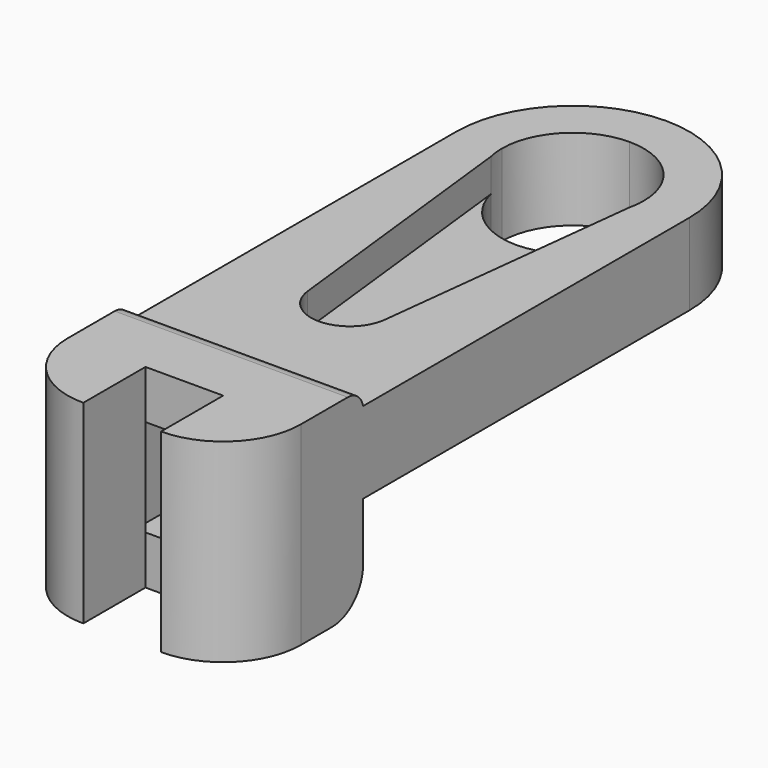
from build123d import *

# Parameters (mm, degrees)
F1_DEPTH      = 4.2
F2_DEPTH      = 2.5
F3_DEPTH      = 5
F3_DEPTH_BACK = 5
F4_W          = 5
F4_H          = 5
F5_DEPTH      = 4
F5_DEPTH_BACK = 4
F6_SIZE       = 2
F7_W          = 4
F7_H          = 2.5
F8_DEPTH      = 25
F9_R          = 2
F11_DEPTH     = 1
F13_DEPTH     = 1
F14_T1_DEPTH  = 16.8989794856


# Not quite as in the source:
# - a fillet or chamfer that OpenCascade refuses, or shapes differently, is made with other operations: its cross-section is extruded or revolved along the edge and cut away or added


with BuildPart() as f1:
    # F0 (on Top) → F1 (new body)
    with BuildSketch(Plane.XY):
        with BuildLine():
            ThreePointArc((6, 14.5), (0, 20.5), (-6, 14.5))
            Line((-6, 14.5), (-3.65, 14.5))
            ThreePointArc((-3.65, 14.5), (-2.5809397513, 17.0809397513), (0, 18.15))
            ThreePointArc((0, 18.15), (2.5809397513, 17.0809397513), (3.65, 14.5))
            Line((3.65, 14.5), (6, 14.5))
        make_face()
        with BuildLine():
            Line((6, -6.5), (-6, -6.5))
            Line((-6, -6.5), (-6, -10.5))
            ThreePointArc((-6, -10.5), (-4.8284271247, -13.3284271247), (-2, -14.5))
            Line((-2, -14.5), (-2, -10.5))
            Line((-2, -10.5), (0, -10.5))
            Line((0, -10.5), (2, -10.5))
            Line((2, -10.5), (2, -14.5))
            ThreePointArc((2, -14.5), (4.8284271247, -13.3284271247), (6, -10.5))
            Line((6, -10.5), (6, -6.5))
        make_face()
        with BuildLine():
            Line((-3.65, 14.5), (-6, 14.5))
            Line((-6, 14.5), (-6, -6.5))
            Line((-6, -6.5), (6, -6.5))
            Line((6, -6.5), (6, 14.5))
            Line((6, 14.5), (3.65, 14.5))
            ThreePointArc((3.65, 14.5), (3.6264789057, 14.0862963062), (3.5562187692, 13.6779245377))
            Line((3.5562187692, 13.6779245377), (1.9871117367, -0.0766868897))
            ThreePointArc((1.9871117367, -0.0766868897), (1.3316580306, -1.3422087286), (0, -1.85))
            ThreePointArc((0, -1.85), (-1.3316580225, -1.3422087358), (-1.9871117342, -0.0766869112))
            Line((-1.9871117342, -0.0766869112), (-3.5562187692, 13.6779245377))
            ThreePointArc((-3.5562187692, 13.6779245377), (-3.6264789057, 14.0862963062), (-3.65, 14.5))
        make_face()
    extrude(amount=F1_DEPTH)

    # F0 (on Top) → F2 (join)
    with BuildSketch(Plane.XY):
        with BuildLine():
            ThreePointArc((0, 10.85), (-2.2717751388, 11.6431594866), (-3.5562187692, 13.6779245377))
            Line((-3.5562187692, 13.6779245377), (-1.9871117342, -0.0766869112))
            ThreePointArc((-1.9871117342, -0.0766869112), (-1.4922087358, 1.4816580225), (0, 2.15))
            Line((0, 2.15), (0, 10.85))
        make_face()
        with BuildLine():
            ThreePointArc((3.5562187692, 13.6779245377), (2.2717751388, 11.6431594866), (0, 10.85))
            Line((0, 10.85), (0, 2.15))
            ThreePointArc((0, 2.15), (1.4142135624, 1.5642135624), (2, 0.15))
            ThreePointArc((2, 0.15), (1.9967753346, 0.0364735127), (1.9871117367, -0.0766868897))
            Line((1.9871117367, -0.0766868897), (3.5562187692, 13.6779245377))
        make_face()
        with BuildLine():
            ThreePointArc((0, 2.15), (-1.4922087358, 1.4816580225), (-1.9871117342, -0.0766869112))
            ThreePointArc((-1.9871117342, -0.0766869112), (-1.3316580225, -1.3422087358), (0, -1.85))
            Line((0, -1.85), (0, 2.15))
        make_face()
        with BuildLine():
            ThreePointArc((2, 0.15), (1.4142135624, 1.5642135624), (0, 2.15))
            Line((0, 2.15), (0, -1.85))
            ThreePointArc((0, -1.85), (1.3316580306, -1.3422087286), (1.9871117367, -0.0766868897))
            ThreePointArc((1.9871117367, -0.0766868897), (1.9967753346, 0.0364735127), (2, 0.15))
        make_face()
    extrude(amount=F2_DEPTH)

    # F0 (on Top) → F3 (join, two sides)
    with BuildSketch(Plane.XY) as f3_sk:
        with BuildLine():
            Line((6, -6.5), (-6, -6.5))
            Line((-6, -6.5), (-6, -10.5))
            ThreePointArc((-6, -10.5), (-4.8284271247, -13.3284271247), (-2, -14.5))
            Line((-2, -14.5), (-2, -10.5))
            Line((-2, -10.5), (0, -10.5))
            Line((0, -10.5), (2, -10.5))
            Line((2, -10.5), (2, -14.5))
            ThreePointArc((2, -14.5), (4.8284271247, -13.3284271247), (6, -10.5))
            Line((6, -10.5), (6, -6.5))
        make_face()
    extrude(amount=F3_DEPTH)
    extrude(f3_sk.sketch, amount=-F3_DEPTH_BACK)

    # F4 (on face) → F5 (cut, two sides)
    with BuildSketch(Plane(origin=(0, -6.5, 0), x_dir=(-1, 0, 0), z_dir=(0, 1, 0))) as f5_sk:
        Rectangle(F4_W, F4_H)
    extrude(amount=-F5_DEPTH, mode=Mode.SUBTRACT)
    extrude(f5_sk.sketch, amount=F5_DEPTH_BACK, mode=Mode.SUBTRACT)

    # F6
    f6_edges = [f1.edges().sort_by_distance(p)[0] for p in [
        (0, -2.5, 2.5),
    ]]
    chamfer(f6_edges, length=F6_SIZE)

    # F7 (on face) → F8 (cut)
    with BuildSketch(Plane.XZ.offset(10.5)):
        with Locations((0, -3.75)):
            Rectangle(F7_W, F7_H)
    extrude(amount=-F8_DEPTH, mode=Mode.SUBTRACT)

    # F9
    f9_edges = [f1.edges().sort_by_distance(p)[0] for p in [
        (4, -6.5, -5),
        (-4, -6.5, -5),
    ]]
    fillet(f9_edges, radius=F9_R)

    # F10 (on face) → F11 (join)
    with BuildSketch(Plane.YZ.offset(-2)):
        with BuildLine():
            Line((-6.5, -2.5), (-10.5, -2.5))
            Line((-10.5, -2.5), (-10.5, -5))
            Line((-10.5, -5), (-8.5, -5))
            ThreePointArc((-8.5, -5), (-7.0857864376, -4.4142135624), (-6.5, -3))
            Line((-6.5, -3), (-6.5, -2.5))
        make_face()
    extrude(amount=F11_DEPTH)

    # F12 (on face) → F13 (join)
    with BuildSketch(Plane(origin=(2, 0, 0), x_dir=(0, -1, 0), z_dir=(-1, 0, 0))):
        with BuildLine():
            Line((10.5, -5), (10.5, -2.5))
            Line((10.5, -2.5), (6.5, -2.5))
            Line((6.5, -2.5), (6.5, -3))
            ThreePointArc((6.5, -3), (7.0857864376, -4.4142135624), (8.5, -5))
            Line((8.5, -5), (10.5, -5))
        make_face()
    extrude(amount=F13_DEPTH)

    # F14: fillet of radius 1 on 1 edges, made by hand

    # F14_s2 → F14_t1 (cut)
    with BuildSketch(Plane.YZ.offset(-8.4494897428)):
        with BuildLine():
            ThreePointArc((-6.5, 4.2), (-6.8473403651, 4.7745966692), (-7.4797958971, 5))
            Line((-7.4797958971, 5), (-6.5, 5))
            Line((-6.5, 5), (-6.5, 4.2))
        make_face()
    extrude(amount=F14_T1_DEPTH, mode=Mode.SUBTRACT)


solid = f1.part
